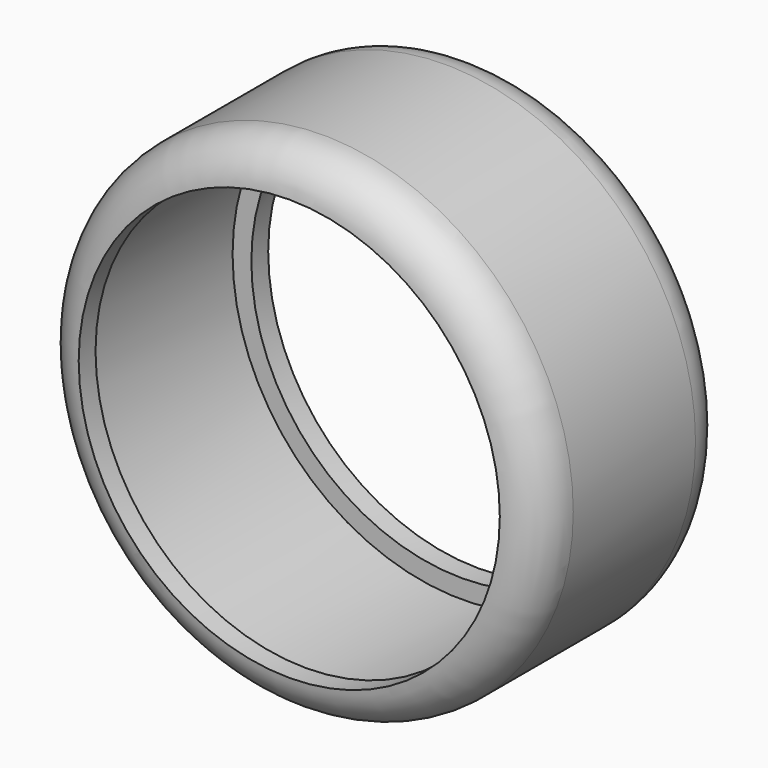
from build123d import *

# Parameters (mm, degrees)
F0_R     = 30.20441
F0_R_2   = 25.4
F2_DEPTH = 28.575
F3_T     = -2.54


# Not quite as in the source:
# - a fillet or chamfer that OpenCascade refuses, or shapes differently, is made with other operations: its cross-section is extruded or revolved along the edge and cut away or added


with BuildPart() as f2:
    # F0 (on Front) → F2 (new body)
    with BuildSketch(Plane.XZ):
        Circle(F0_R)
        Circle(F0_R_2, mode=Mode.SUBTRACT)
    extrude(amount=F2_DEPTH)

    # F3
    f3_openings = [f2.faces().sort_by_distance(p)[0] for p in [
        (-25.4, -14.2875, 0),
    ]]
    offset(amount=F3_T, openings=f3_openings)

    # F4: fillet of radius 5.08 on 2 edges, made by hand

    # F4_s1 → F4_t2 (revolve, cut)
    with BuildSketch(Plane.XY):
        with BuildLine():
            ThreePointArc((30.20441, -5.072519113), (28.8126614285, -1.5792110247), (25.4, 0))
            Line((25.4, 0), (30.20441, 0))
            Line((30.20441, 0), (30.20441, -5.072519113))
        make_face()
    revolve(axis=Axis((0, 0, 0), (0, -1, 0)), mode=Mode.SUBTRACT)

    # F4_s3 → F4_t4 (revolve, cut)
    with BuildSketch(Plane.XY):
        with BuildLine():
            ThreePointArc((30.20441, -23.502480887), (28.8126614285, -26.9957889753), (25.4, -28.575))
            Line((25.4, -28.575), (30.20441, -28.575))
            Line((30.20441, -28.575), (30.20441, -23.502480887))
        make_face()
    revolve(axis=Axis((0, -28.575, 0), (0, -1, 0)), mode=Mode.SUBTRACT)


solid = f2.part
